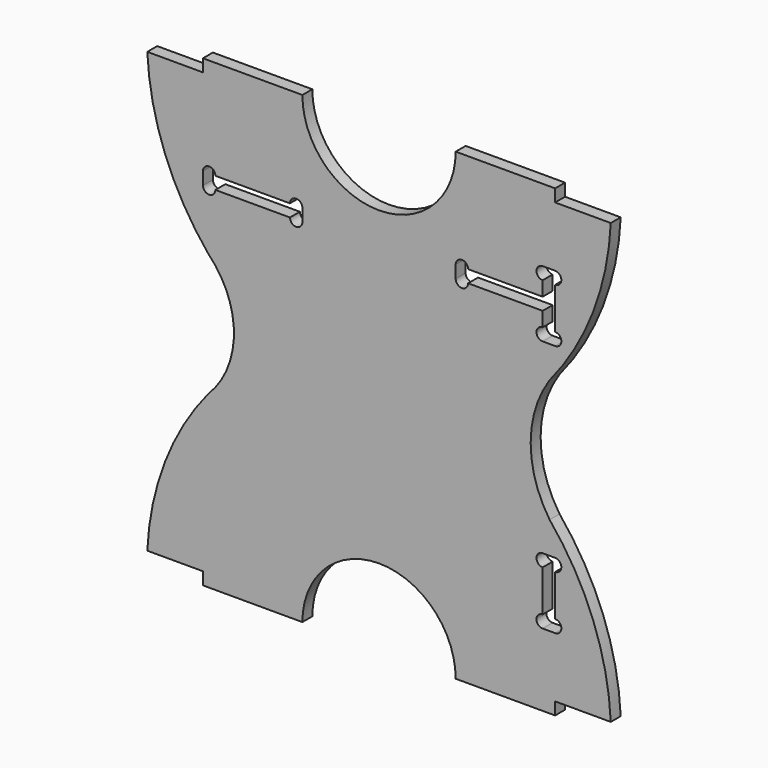
from build123d import *

# Parameters (mm, degrees)
F2_DEPTH  = 19.05
F3_W      = 85.725
F3_H      = 19.05
F3_R      = 117.475
F4_DEPTH  = 25.4
F5_W      = 152.4
F5_H      = 19.05
F6_DEPTH  = 25.4
F8_DEPTH  = 25.4
F9_W      = 19.05
F9_H      = 101.6
F10_DEPTH = 25.4
F12_DEPTH = 25.4


# Not quite as in the source:
# - a variable given as a bare number and used for a length is read in inches; the dataset says mm whatever the document's units were


with BuildPart() as f2:
    # F1 (on Front) → F2 (new body)
    with BuildSketch(Plane.XZ):
        with BuildLine():
            Line((355.6, 355.6), (203.2, 355.6))
            Line((203.2, 355.6), (-203.2, 355.6))
            Line((-203.2, 355.6), (-355.6, 355.6))
            ThreePointArc((-355.6, 355.6), (-331.3431214209, 216.6595631931), (-261.4423933195, 94.1576066805))
            ThreePointArc((-261.4423933195, 94.1576066805), (-222.3790342141, 0), (-261.4423933195, -94.1576066805))
            ThreePointArc((-261.4423933195, -94.1576066805), (-331.3431214209, -216.6595631931), (-355.6, -355.6))
            Line((-355.6, -355.6), (-203.2, -355.6))
            Line((-203.2, -355.6), (203.2, -355.6))
            Line((203.2, -355.6), (355.6, -355.6))
            ThreePointArc((355.6, -355.6), (331.3431214209, -216.6595631931), (261.4423933195, -94.1576066805))
            ThreePointArc((261.4423933195, -94.1576066805), (232.4074653208, 0), (261.4423933195, 94.1576066805))
            ThreePointArc((261.4423933195, 94.1576066805), (331.3431214209, 216.6595631931), (355.6, 355.6))
        make_face()
    extrude(amount=F2_DEPTH)

    # F3 (on face) → F4 (cut)
    with BuildSketch(Plane.XZ.offset(19.05)):
        with Locations((-312.7375, 346.075)):
            Rectangle(F3_W, F3_H)
        with Locations((312.7375, 346.075)):
            Rectangle(F3_W, F3_H)
        with Locations((312.7375, -346.075)):
            Rectangle(F3_W, F3_H)
        with Locations((-312.7375, -346.075)):
            Rectangle(F3_W, F3_H)
        with Locations((0, 355.6)):
            Circle(F3_R)
        with Locations((0, -355.6)):
            Circle(F3_R)
    extrude(amount=-F4_DEPTH, mode=Mode.SUBTRACT)

    # F5 (on face) → F6 (cut)
    with BuildSketch(Plane.XZ.offset(19.05)):
        with Locations((-193.675, 193.675)):
            Rectangle(F5_W, F5_H)
        with Locations((193.675, 193.675)):
            Rectangle(F5_W, F5_H)
    extrude(amount=-F6_DEPTH, mode=Mode.SUBTRACT)

    # F7 (on face) → F8 (cut)
    with BuildSketch(Plane.XZ.offset(19.05)):
        with BuildLine():
            Line((-250.825, 184.15), (-250.825, 203.2))
            ThreePointArc((-250.825, 203.2), (-260.35, 212.725), (-269.875, 203.2))
            Line((-269.875, 203.2), (-269.875, 184.15))
            ThreePointArc((-269.875, 184.15), (-260.35, 174.625), (-250.825, 184.15))
        make_face()
        with BuildLine():
            ThreePointArc((-117.475, 203.2), (-127, 212.725), (-136.525, 203.2))
            Line((-136.525, 203.2), (-136.525, 184.15))
            ThreePointArc((-136.525, 184.15), (-127, 174.625), (-117.475, 184.15))
            Line((-117.475, 184.15), (-117.475, 203.2))
        make_face()
        with BuildLine():
            Line((117.475, 203.2), (117.475, 184.15))
            ThreePointArc((117.475, 184.15), (127, 174.625), (136.525, 184.15))
            Line((136.525, 184.15), (136.525, 203.2))
            ThreePointArc((136.525, 203.2), (127, 212.725), (117.475, 203.2))
        make_face()
        with BuildLine():
            ThreePointArc((269.875, 203.2), (260.35, 212.725), (250.825, 203.2))
            Line((250.825, 203.2), (250.825, 184.15))
            ThreePointArc((250.825, 184.15), (260.35, 174.625), (269.875, 184.15))
            Line((269.875, 184.15), (269.875, 203.2))
        make_face()
    extrude(amount=-F8_DEPTH, mode=Mode.SUBTRACT)

    # F9 (on face) → F10 (cut)
    with BuildSketch(Plane.XZ.offset(19.05)):
        with Locations((260.35, 193.675)):
            Rectangle(F9_W, F9_H)
        with Locations((260.35, -193.675)):
            Rectangle(F9_W, F9_H)
    extrude(amount=-F10_DEPTH, mode=Mode.SUBTRACT)

    # F11 (on face) → F12 (cut)
    with BuildSketch(Plane.XZ.offset(19.05)):
        with BuildLine():
            Line((269.875, 244.475), (250.825, 244.475))
            ThreePointArc((250.825, 244.475), (241.3, 234.95), (250.825, 225.425))
            Line((250.825, 225.425), (269.875, 225.425))
            ThreePointArc((269.875, 225.425), (279.4, 234.95), (269.875, 244.475))
        make_face()
        with BuildLine():
            ThreePointArc((269.875, 142.875), (279.4, 152.4), (269.875, 161.925))
            Line((269.875, 161.925), (250.825, 161.925))
            ThreePointArc((250.825, 161.925), (241.3, 152.4), (250.825, 142.875))
            Line((250.825, 142.875), (269.875, 142.875))
        make_face()
        with BuildLine():
            Line((269.875, -142.875), (250.825, -142.875))
            ThreePointArc((250.825, -142.875), (241.3, -152.4), (250.825, -161.925))
            Line((250.825, -161.925), (269.875, -161.925))
            ThreePointArc((269.875, -161.925), (279.4, -152.4), (269.875, -142.875))
        make_face()
        with BuildLine():
            ThreePointArc((250.825, -225.425), (241.3, -234.95), (250.825, -244.475))
            Line((250.825, -244.475), (269.875, -244.475))
            ThreePointArc((269.875, -244.475), (279.4, -234.95), (269.875, -225.425))
            Line((269.875, -225.425), (250.825, -225.425))
        make_face()
    extrude(amount=-F12_DEPTH, mode=Mode.SUBTRACT)


solid = f2.part
